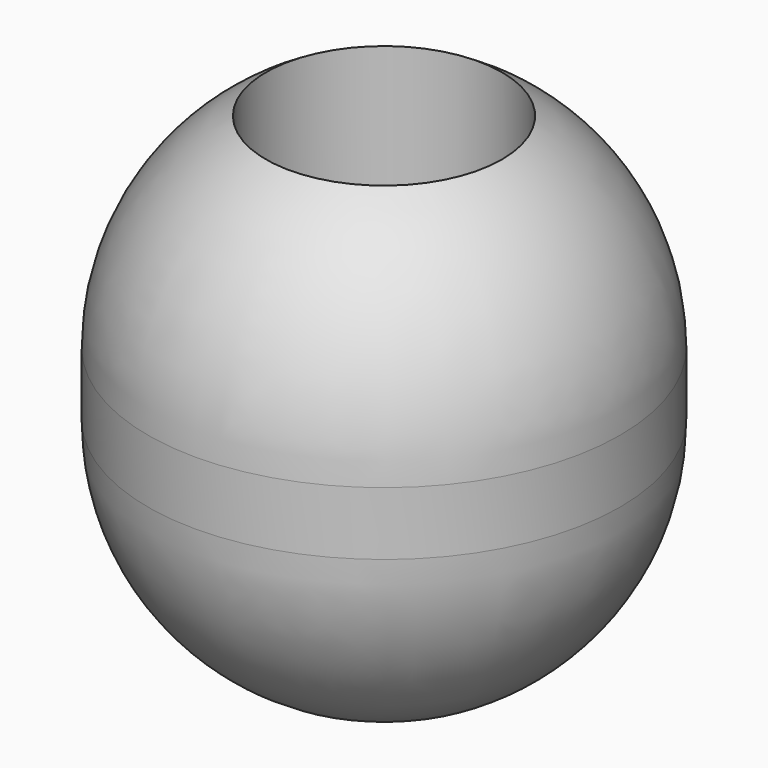
from build123d import *

# Parameters (mm, degrees)
F1_R     = 25.4
F2_DEPTH = 101.6
F0_R     = 50.8
F3_DEPTH = 101.6
F4_R     = 25.4
F5_DEPTH = 101.601


# Not quite as in the source:
# - a fillet or chamfer that OpenCascade refuses, or shapes differently, is made with other operations: its cross-section is extruded or revolved along the edge and cut away or added


with BuildPart() as f2:
    # F1 (on face) → F2 (new body)
    with BuildSketch(Plane.XY):
        Circle(F1_R)
    extrude(amount=F2_DEPTH)

    # F0 (on Top) → F3 (join)
    with BuildSketch(Plane.XY):
        Circle(F0_R)
    extrude(amount=F3_DEPTH)

    # F4 (on face) → F5 (cut, through all)
    with BuildSketch(Plane(origin=(0, 0, 0), x_dir=(1, 0, 0), z_dir=(0, 0, -1))):
        Circle(F4_R)
    extrude(amount=-F5_DEPTH, mode=Mode.SUBTRACT)

    # F6: fillet of radius 50.79746 on 2 edges, made by hand

    # F6_s1 → F6_t2 (revolve, cut)
    with BuildSketch(Plane.XZ):
        with BuildLine():
            ThreePointArc((50.8, 57.6073759819), (43.9940641888, 83.0067409739), (25.4, 101.6))
            Line((25.4, 101.6), (50.8, 101.6))
            Line((50.8, 101.6), (50.8, 57.6073759819))
        make_face()
    revolve(axis=Axis((0, 0, 101.6), (0, 0, 1)), mode=Mode.SUBTRACT)

    # F6_s3 → F6_t4 (revolve, cut)
    with BuildSketch(Plane.XZ):
        with BuildLine():
            ThreePointArc((50.8, 43.9926240181), (43.9940641888, 18.5932590261), (25.4, 0))
            Line((25.4, 0), (50.8, 0))
            Line((50.8, 0), (50.8, 43.9926240181))
        make_face()
    revolve(axis=Axis((0, 0, 0), (0, 0, 1)), mode=Mode.SUBTRACT)


solid = f2.part
